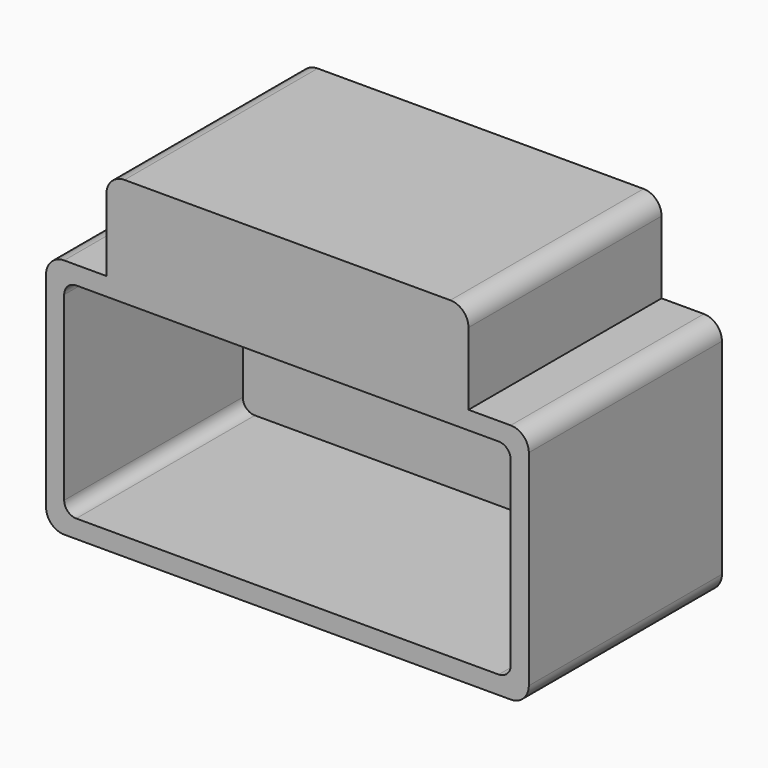
from build123d import *

# Parameters (mm, degrees)
F1_DEPTH = 50.8
F2_T     = 3.81
F3_R     = 2.54
F4_DEPTH = 50.8


# Not quite as in the source:
# - a shell that OpenCascade refuses in one call is made with other operations: the cavity is built on its own and cut out


with BuildPart() as f1:
    # F0 (on Front) → F1 (new body)
    with BuildSketch(Plane.XZ):
        with BuildLine():
            ThreePointArc((50.8, 21.59), (49.6840768363, 24.2840768363), (46.99, 25.4))
            Line((46.99, 25.4), (38.1, 25.4))
            Line((38.1, 25.4), (-38.1, 25.4))
            Line((-38.1, 25.4), (-46.99, 25.4))
            ThreePointArc((-46.99, 25.4), (-49.6840768363, 24.2840768363), (-50.8, 21.59))
            Line((-50.8, 21.59), (-50.8, -21.59))
            ThreePointArc((-50.8, -21.59), (-49.6840768363, -24.2840768363), (-46.99, -25.4))
            Line((-46.99, -25.4), (46.99, -25.4))
            ThreePointArc((46.99, -25.4), (49.6840768363, -24.2840768363), (50.8, -21.59))
            Line((50.8, -21.59), (50.8, 21.59))
        make_face()
    extrude(amount=F1_DEPTH)

    # F2: shell of thickness 3.81, made by hand


with BuildPart() as f2_core1:
    # F2_t2: copy of F1
    add(f1.part)

    # the walls: a layer under each face that stays
    f2_faces = [f2_core1.faces().sort_by_distance(p)[0] for p in [
        (0, -25.4, -25.4),
        (-50.8, -25.4, 0),
        (0, 0, 0),
        (0, -25.4, 25.4),
        (50.8, -25.4, 0),
    ]]
    thicken(f2_faces, amount=-F2_T, mode=Mode.SUBTRACT)


with BuildPart() as f1_1:
    add(f1.part)

    # what is left inside the walls is the cavity
    f2_cavity = [f2_core1.part.solids().sort_by_distance(p)[0] for p in [
        (0, -35.136667, -21.5519),
    ]]
    add(f2_cavity, mode=Mode.SUBTRACT)

    # F3
    f3_edges = [f1_1.edges().sort_by_distance(p)[0] for p in [
        (-46.99, -27.305, 21.59),
        (-46.99, -27.305, -21.59),
        (46.99, -27.305, -21.59),
        (46.99, -27.305, 21.59),
    ]]
    fillet(f3_edges, radius=F3_R)

    # F0 (on Front) → F4 (join)
    with BuildSketch(Plane.XZ):
        with BuildLine():
            Line((-38.1, 25.4), (38.1, 25.4))
            Line((38.1, 25.4), (38.1, 40.64))
            ThreePointArc((38.1, 40.64), (36.9840768363, 43.3340768363), (34.29, 44.45))
            Line((34.29, 44.45), (0, 44.45))
            Line((0, 44.45), (-34.29, 44.45))
            ThreePointArc((-34.29, 44.45), (-36.9840768363, 43.3340768363), (-38.1, 40.64))
            Line((-38.1, 40.64), (-38.1, 25.4))
        make_face()
    extrude(amount=F4_DEPTH)


solid = f1_1.part
